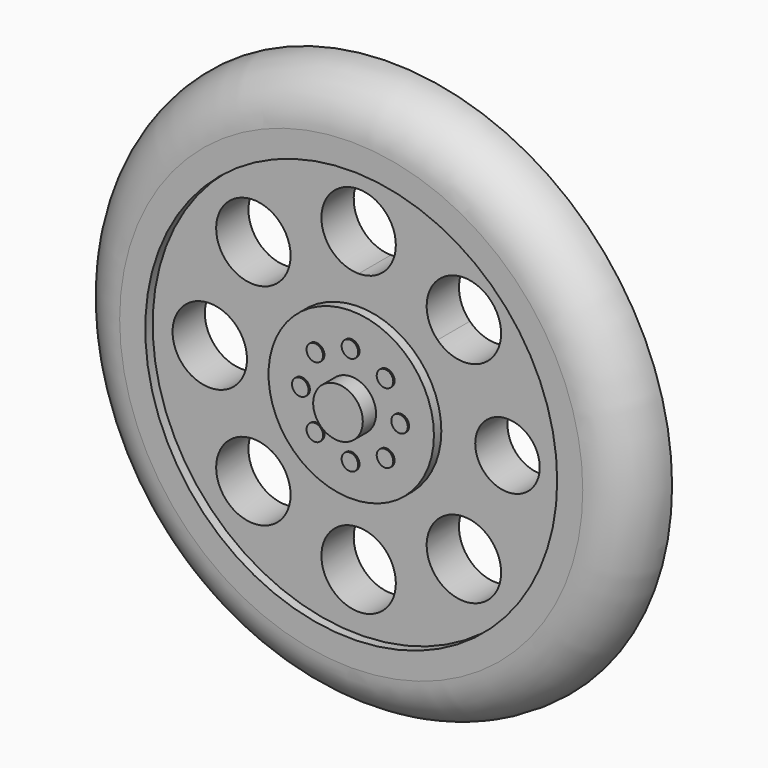
from build123d import *

# Parameters (mm, degrees)
F0_R      = 17
F1_DEPTH  = 3
F3_R      = 2.99999
F5_R      = 12.4526743877
F6_DEPTH  = 0.5588
F7_R      = 5
F8_DEPTH  = 1.143
F10_R     = 2.25
F11_DEPTH = 25.4
F13_DEPTH = 0.1
F14_R     = 1.5
F15_DEPTH = 1


# Not quite as in the source:
# - a fillet or chamfer is up to 0.001 mm smaller than in the source, because OpenCascade refuses the exact size


with BuildPart() as f1:
    # F0 (on Front) → F1 (new body)
    with BuildSketch(Plane.XZ):
        Circle(F0_R)
    extrude(amount=F1_DEPTH)

    # F3 (radius 3 in the source; OpenCascade refuses exactly that, so slightly less here)
    f3_edges = [f1.edges().sort_by_distance(p)[0] for p in [
        (-17, -3, 0),
    ]]
    fillet(f3_edges, radius=F3_R)

    # F5 (on face) → F6 (cut)
    with BuildSketch(Plane.XZ.offset(3)):
        Circle(F5_R)
    extrude(amount=-F6_DEPTH, mode=Mode.SUBTRACT)

    # F7 (on face) → F8 (join)
    with BuildSketch(Plane.XZ.offset(3)):
        Circle(F7_R)
    extrude(amount=-F8_DEPTH)

    # F10 (on face) → F11 (cut)
    with BuildSketch(Plane.XZ.offset(3)):
        with BuildLine():
            ThreePointArc((8.6139610307, -6.3639610307), (7.2249987535, -4.2852320825), (4.772970773, -4.772970773))
            ThreePointArc((4.772970773, -4.772970773), (5.5029233079, -8.4426899788), (8.6139610307, -6.3639610307))
        make_face()
        with BuildLine():
            ThreePointArc((2.25, -9), (1.5909902577, -7.4090097423), (0, -6.75))
            ThreePointArc((0, -6.75), (-1.5909902577, -10.5909902577), (2.25, -9))
        make_face()
        with BuildLine():
            ThreePointArc((-4.1139610307, -6.3639610307), (-4.2852320825, -5.5029233079), (-4.772970773, -4.772970773))
            ThreePointArc((-4.772970773, -4.772970773), (-8.4426899788, -7.2249987535), (-4.1139610307, -6.3639610307))
        make_face()
        with BuildLine():
            ThreePointArc((10.9506839843, 0), (9, 1.9506839843), (7.0493160157, 0))
            ThreePointArc((7.0493160157, 0), (9, -1.9506839843), (10.9506839843, 0))
        make_face()
        with Locations((-9, 0)):
            Circle(F10_R)
        with BuildLine():
            ThreePointArc((-4.1139610307, 6.3639610307), (-8.4426899788, 7.2249987535), (-4.772970773, 4.772970773))
            ThreePointArc((-4.772970773, 4.772970773), (-4.2852320825, 5.5029233079), (-4.1139610307, 6.3639610307))
        make_face()
        with BuildLine():
            ThreePointArc((2.25, 9), (-1.5909902577, 10.5909902577), (0, 6.75))
            ThreePointArc((0, 6.75), (1.5909902577, 7.4090097423), (2.25, 9))
        make_face()
        with BuildLine():
            ThreePointArc((8.6139610307, 6.3639610307), (5.5029233079, 8.4426899788), (4.772970773, 4.772970773))
            ThreePointArc((4.772970773, 4.772970773), (7.2249987535, 4.2852320825), (8.6139610307, 6.3639610307))
        make_face()
    extrude(amount=-F11_DEPTH, mode=Mode.SUBTRACT)

    # F12 (on face) → F13 (join)
    with BuildSketch(Plane.XZ.offset(3)):
        with BuildLine():
            Line((-2.1213203436, 2.1213203436), (-1.767766953, 1.767766953))
            ThreePointArc((-1.767766953, 1.767766953), (-1.6593805773, 1.9299786274), (-1.6213203436, 2.1213203436))
            ThreePointArc((-1.6213203436, 2.1213203436), (-1.9299786274, 2.5832601098), (-2.4748737342, 2.4748737342))
            Line((-2.4748737342, 2.4748737342), (-2.1213203436, 2.1213203436))
        make_face()
        with BuildLine():
            ThreePointArc((-2.4748737342, 2.4748737342), (-2.4748737342, 1.767766953), (-1.767766953, 1.767766953))
            Line((-1.767766953, 1.767766953), (-2.1213203436, 2.1213203436))
            Line((-2.1213203436, 2.1213203436), (-2.4748737342, 2.4748737342))
        make_face()
        with BuildLine():
            Line((0, 3), (0, 3.5))
            ThreePointArc((0, 3.5), (-0.5, 3), (0, 2.5))
            Line((0, 2.5), (0, 3))
        make_face()
        with BuildLine():
            ThreePointArc((0.5, 3), (0.3535533906, 3.3535533906), (0, 3.5))
            Line((0, 3.5), (0, 3))
            Line((0, 3), (0, 2.5))
            ThreePointArc((0, 2.5), (0.3535533906, 2.6464466094), (0.5, 3))
        make_face()
        with BuildLine():
            ThreePointArc((2.6213203436, -2.1213203436), (2.3126620597, -1.6593805773), (1.767766953, -1.767766953))
            Line((1.767766953, -1.767766953), (2.1213203436, -2.1213203436))
            Line((2.1213203436, -2.1213203436), (2.4748737342, -2.4748737342))
            ThreePointArc((2.4748737342, -2.4748737342), (2.5832601098, -2.3126620597), (2.6213203436, -2.1213203436))
        make_face()
        with BuildLine():
            Line((2.1213203436, -2.1213203436), (1.767766953, -1.767766953))
            ThreePointArc((1.767766953, -1.767766953), (1.767766953, -2.4748737342), (2.4748737342, -2.4748737342))
            Line((2.4748737342, -2.4748737342), (2.1213203436, -2.1213203436))
        make_face()
        with BuildLine():
            ThreePointArc((-3.5, 0), (-3, -0.5), (-2.5, 0))
            Line((-2.5, 0), (-3, 0))
            Line((-3, 0), (-3.5, 0))
        make_face()
        with BuildLine():
            Line((-3, 0), (-2.5, 0))
            ThreePointArc((-2.5, 0), (-3, 0.5), (-3.5, 0))
            Line((-3.5, 0), (-3, 0))
        make_face()
        with BuildLine():
            Line((-2.1213203436, -2.1213203436), (-1.767766953, -1.767766953))
            ThreePointArc((-1.767766953, -1.767766953), (-2.4748737342, -1.767766953), (-2.4748737342, -2.4748737342))
            Line((-2.4748737342, -2.4748737342), (-2.1213203436, -2.1213203436))
        make_face()
        with BuildLine():
            ThreePointArc((-1.6213203436, -2.1213203436), (-1.6593805773, -1.9299786274), (-1.767766953, -1.767766953))
            Line((-1.767766953, -1.767766953), (-2.1213203436, -2.1213203436))
            Line((-2.1213203436, -2.1213203436), (-2.4748737342, -2.4748737342))
            ThreePointArc((-2.4748737342, -2.4748737342), (-1.9299786274, -2.5832601098), (-1.6213203436, -2.1213203436))
        make_face()
        with BuildLine():
            ThreePointArc((0.5, -3), (0.3535533906, -2.6464466094), (0, -2.5))
            Line((0, -2.5), (0, -3))
            Line((0, -3), (0, -3.5))
            ThreePointArc((0, -3.5), (0.3535533906, -3.3535533906), (0.5, -3))
        make_face()
        with BuildLine():
            Line((0, -3), (0, -2.5))
            ThreePointArc((0, -2.5), (-0.5, -3), (0, -3.5))
            Line((0, -3.5), (0, -3))
        make_face()
        with BuildLine():
            Line((3, 0), (2.5, 0))
            ThreePointArc((2.5, 0), (3, -0.5), (3.5, 0))
            Line((3.5, 0), (3, 0))
        make_face()
        with BuildLine():
            ThreePointArc((3.5, 0), (3, 0.5), (2.5, 0))
            Line((2.5, 0), (3, 0))
            Line((3, 0), (3.5, 0))
        make_face()
        with BuildLine():
            Line((2.1213203436, 2.1213203436), (1.767766953, 1.767766953))
            ThreePointArc((1.767766953, 1.767766953), (2.3126620597, 1.6593805773), (2.6213203436, 2.1213203436))
            ThreePointArc((2.6213203436, 2.1213203436), (2.5832601098, 2.3126620597), (2.4748737342, 2.4748737342))
            Line((2.4748737342, 2.4748737342), (2.1213203436, 2.1213203436))
        make_face()
        with BuildLine():
            ThreePointArc((2.4748737342, 2.4748737342), (1.767766953, 2.4748737342), (1.767766953, 1.767766953))
            Line((1.767766953, 1.767766953), (2.1213203436, 2.1213203436))
            Line((2.1213203436, 2.1213203436), (2.4748737342, 2.4748737342))
        make_face()
    extrude(amount=F13_DEPTH)

    # F14 (on face) → F15 (join)
    with BuildSketch(Plane.XZ.offset(3)):
        Circle(F14_R)
    extrude(amount=F15_DEPTH)


solid = f1.part
